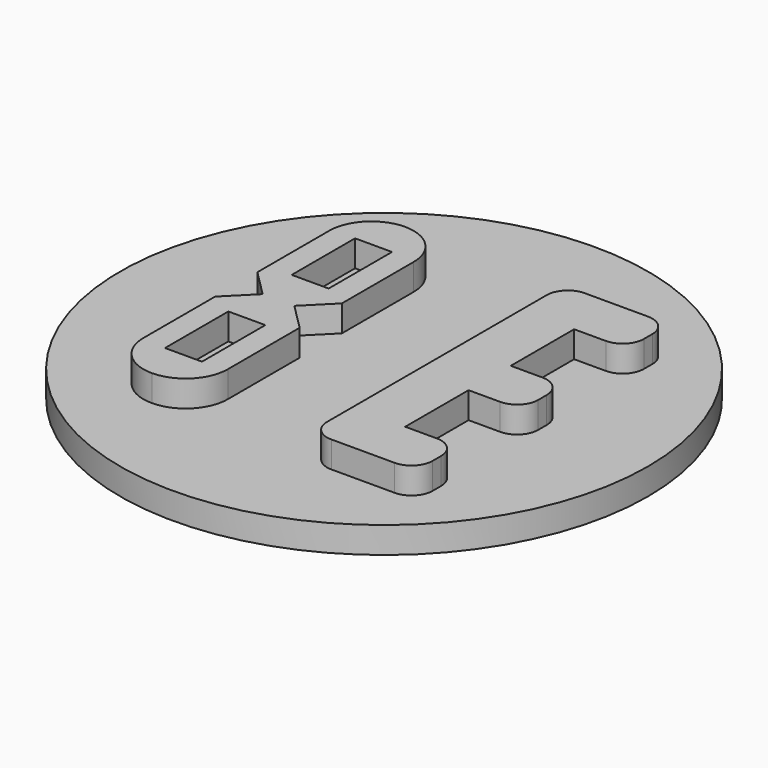
from build123d import *

# Parameters (mm, degrees)
F0_R     = 63.5
F1_DEPTH = 6.35
F3_DEPTH = 6.35
F4_W     = 12.7
F4_H     = 12.7
F5_DEPTH = 6.35
F6_R     = 10.15999
F7_R     = 5.08
F8_W     = 8.89
F8_H     = 19.05
F9_DEPTH = 6.35


# Not quite as in the source:
# - a fillet or chamfer is up to 0.001 mm smaller than in the source, because OpenCascade refuses the exact size
# - a feature names something its author has since deleted; it is built from what else it names


with BuildPart() as f1:
    # F0 (on Top) → F1 (new body)
    with BuildSketch(Plane.XY):
        Circle(F0_R)
    extrude(amount=F1_DEPTH)

    # F2 (on face) → F3 (join)
    with BuildSketch(Plane.XY.offset(6.35)):
        Polygon((-21.59, 0), (-25.4, 0), (-29.21, 0), (-35.56, -6.35), (-35.56, -38.1), (-15.24, -38.1), (-15.24, -6.35), align=None)
        Polygon((-29.21, 0), (-25.4, 0), (-21.59, 0), (-15.24, 6.35), (-15.24, 38.1), (-35.56, 38.1), (-35.56, 6.35), align=None)
    extrude(amount=F3_DEPTH)

    # F4 (on face) → F5 (join)
    with BuildSketch(Plane.XY.offset(6.35)):
        Polygon((12.7, 38.1), (12.7, 0), (12.7, -38.1), (25.4, -38.1), (25.4, -25.4), (25.4, -6.35), (25.4, 0), (25.4, 6.35), (25.4, 25.4), (25.4, 38.1), align=None)
        with Locations((31.75, 31.75)):
            Rectangle(F4_W, F4_H)
        with Locations((31.75, -31.75)):
            Rectangle(F4_W, F4_H)
        Polygon((38.1, 6.35), (25.4, 6.35), (25.4, 0), (25.4, -6.35), (38.1, -6.35), align=None)
    extrude(amount=F5_DEPTH)

    # F6 (radius 10.16 in the source; OpenCascade refuses exactly that, so slightly less here)
    f6_edges = [f1.edges().sort_by_distance(p)[0] for p in [
        (-35.56, -38.1, 9.525),
        (-15.24, -38.1, 9.525),
        (-15.24, 38.1, 9.525),
        (-35.56, 38.1, 9.525),
    ]]
    fillet(f6_edges, radius=F6_R)

    # F7
    f7_edges = [f1.edges().sort_by_distance(p)[0] for p in [
        (38.1, 6.35, 9.525),
        (38.1, -6.35, 9.525),
        (38.1, -38.1, 9.525),
        (38.1, -25.4, 9.525),
        (38.1, 25.4, 9.525),
        (38.1, 38.1, 9.525),
        (12.7, 38.1, 9.525),
        (12.7, -38.1, 9.525),
    ]]
    fillet(f7_edges, radius=F7_R)

    # F8 (on face) → F9 (cut)
    with BuildSketch(Plane.XY.offset(12.7)):
        Polygon((-29.845, -28.575), (-20.955, -28.575), (-20.955, -9.525), (-25.4, -9.525), (-29.845, -9.525), align=None)
        with Locations((-25.4, 19.05)):
            Rectangle(F8_W, F8_H)
    extrude(amount=-F9_DEPTH, mode=Mode.SUBTRACT)


solid = f1.part
